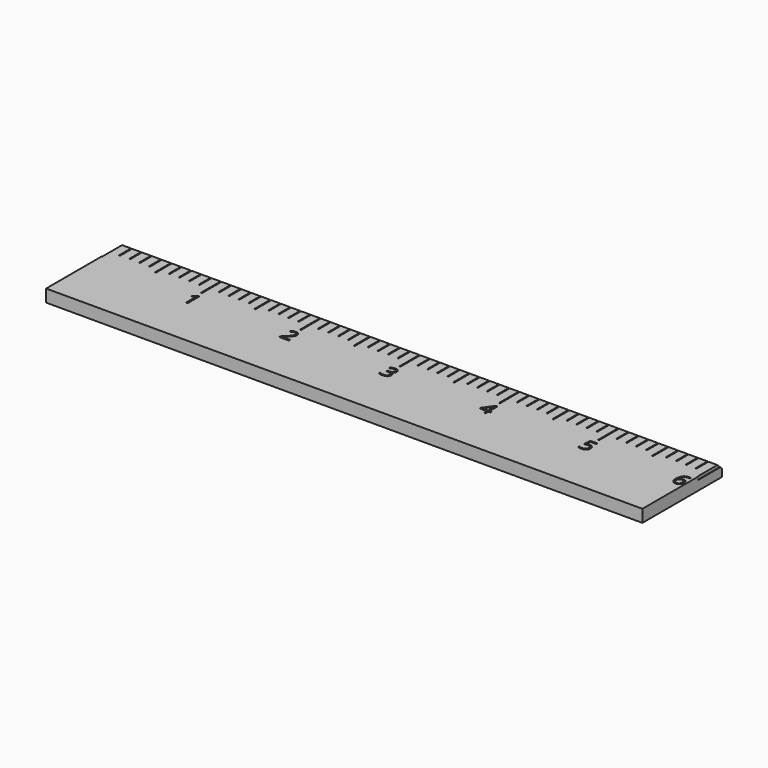
from build123d import *

# Parameters (mm, degrees)
F0_W          = 152.4
F0_H          = 25.4
F1_DEPTH      = 3.175
F2_W          = 0.254
F2_H          = 7.62
F2_H_2        = 5.08
F2_H_3        = 6.35
F3_TEXT_SIZE  = 5.2916666667
F4_DEPTH      = 0.762
F5_T3_DEPTH   = 8.8180747894
F5_T6_DEPTH   = 8.8180747894
F5_T9_DEPTH   = 8.8180747894
F5_T12_DEPTH  = 8.8180747894
F5_T15_DEPTH  = 8.8180747894
F5_T18_DEPTH  = 8.8180747894
F5_T21_DEPTH  = 8.8180747894
F5_T24_DEPTH  = 8.8180747894
F5_T27_DEPTH  = 8.8180747894
F5_T30_DEPTH  = 8.8180747894
F5_T33_DEPTH  = 8.8180747894
F5_T36_DEPTH  = 8.8180747894
F5_T39_DEPTH  = 8.8180747894
F5_T42_DEPTH  = 8.8180747894
F5_T45_DEPTH  = 8.8180747894
F5_T48_DEPTH  = 8.8180747894
F5_T51_DEPTH  = 8.8180747894
F5_T54_DEPTH  = 8.8180747894
F5_T57_DEPTH  = 8.8180747894
F5_T60_DEPTH  = 8.8180747894
F5_T63_DEPTH  = 8.8180747894
F5_T66_DEPTH  = 8.8180747894
F5_T69_DEPTH  = 8.8180747894
F5_T72_DEPTH  = 8.8180747894
F5_T75_DEPTH  = 8.8180747894
F5_T78_DEPTH  = 8.8180747894
F5_T81_DEPTH  = 8.8180747894
F5_T84_DEPTH  = 8.8180747894
F5_T87_DEPTH  = 8.8180747894
F5_T90_DEPTH  = 8.8180747894
F5_T93_DEPTH  = 8.8180747894
F5_T96_DEPTH  = 8.8180747894
F5_T99_DEPTH  = 8.8180747894
F5_T102_DEPTH = 8.8180747894
F5_T105_DEPTH = 8.8180747894
F5_T108_DEPTH = 8.8180747894
F5_T111_DEPTH = 8.8180747894
F5_T114_DEPTH = 8.8180747894
F5_T117_DEPTH = 8.8180747894
F5_T120_DEPTH = 8.8180747894
F5_T123_DEPTH = 8.8180747894
F5_T126_DEPTH = 8.8180747894
F5_T129_DEPTH = 8.8180747894
F5_T132_DEPTH = 8.8180747894
F5_T135_DEPTH = 8.8180747894
F5_T138_DEPTH = 8.8180747894
F5_T141_DEPTH = 8.8180747894
F5_T144_DEPTH = 8.8180747894
F5_T147_DEPTH = 8.8180747894
F5_T150_DEPTH = 8.8180747894
F5_T153_DEPTH = 8.8180747894
F5_T156_DEPTH = 8.8180747894
F5_T159_DEPTH = 8.8180747894
F5_T162_DEPTH = 8.8180747894
F5_T165_DEPTH = 8.8180747894
F5_T168_DEPTH = 8.8180747894
F5_T171_DEPTH = 8.8180747894
F5_T174_DEPTH = 8.8180747894
F5_T177_DEPTH = 8.8180747894
F5_T180_DEPTH = 8.8180747894


# Not quite as in the source:
# - a fillet or chamfer that OpenCascade refuses, or shapes differently, is made with other operations: its cross-section is extruded or revolved along the edge and cut away or added
# - Text() gives the source's letters only with a copy of the font that has no kerning and outlines rounded to 1/6400 em; it was checked with that copy


with BuildPart() as f1:
    # F0 (on Top) → F1 (new body)
    with BuildSketch(Plane.XY):
        Rectangle(F0_W, F0_H)
    extrude(amount=F1_DEPTH)

    # F2 (on face) + F3 (on face) → F4 (cut)
    with BuildSketch(Plane.XY.offset(3.175)):
        with Locations((-76.2, 8.89)):
            Rectangle(F2_W, F2_H)
        with Locations((-73.66, 10.16)):
            Rectangle(F2_W, F2_H_2)
        with Locations((-71.12, 10.16)):
            Rectangle(F2_W, F2_H_2)
        with Locations((-68.58, 10.16)):
            Rectangle(F2_W, F2_H_2)
        with Locations((-66.04, 10.16)):
            Rectangle(F2_W, F2_H_2)
        with Locations((-63.5, 9.525)):
            Rectangle(F2_W, F2_H_3)
        with Locations((-60.96, 10.16)):
            Rectangle(F2_W, F2_H_2)
        with Locations((-58.42, 10.16)):
            Rectangle(F2_W, F2_H_2)
        with Locations((-55.88, 10.16)):
            Rectangle(F2_W, F2_H_2)
        with Locations((-53.34, 10.16)):
            Rectangle(F2_W, F2_H_2)
        with Locations((-50.8, 8.89)):
            Rectangle(F2_W, F2_H)
        with Locations((-45.72, 10.16)):
            Rectangle(F2_W, F2_H_2)
        with Locations((-48.26, 10.16)):
            Rectangle(F2_W, F2_H_2)
        with Locations((-33.02, 10.16)):
            Rectangle(F2_W, F2_H_2)
        with Locations((-35.56, 10.16)):
            Rectangle(F2_W, F2_H_2)
        with Locations((-30.48, 10.16)):
            Rectangle(F2_W, F2_H_2)
        with Locations((-38.1, 9.525)):
            Rectangle(F2_W, F2_H_3)
        with Locations((-43.18, 10.16)):
            Rectangle(F2_W, F2_H_2)
        with Locations((-40.64, 10.16)):
            Rectangle(F2_W, F2_H_2)
        with Locations((-25.4, 8.89)):
            Rectangle(F2_W, F2_H)
        with Locations((-27.94, 10.16)):
            Rectangle(F2_W, F2_H_2)
        with Locations((-20.32, 10.16)):
            Rectangle(F2_W, F2_H_2)
        with Locations((-22.86, 10.16)):
            Rectangle(F2_W, F2_H_2)
        with Locations((-7.62, 10.16)):
            Rectangle(F2_W, F2_H_2)
        with Locations((-10.16, 10.16)):
            Rectangle(F2_W, F2_H_2)
        with Locations((-5.08, 10.16)):
            Rectangle(F2_W, F2_H_2)
        with Locations((-12.7, 9.525)):
            Rectangle(F2_W, F2_H_3)
        with Locations((-17.78, 10.16)):
            Rectangle(F2_W, F2_H_2)
        with Locations((-15.24, 10.16)):
            Rectangle(F2_W, F2_H_2)
        with Locations((0, 8.89)):
            Rectangle(F2_W, F2_H)
        with Locations((-2.54, 10.16)):
            Rectangle(F2_W, F2_H_2)
        with Locations((5.08, 10.16)):
            Rectangle(F2_W, F2_H_2)
        with Locations((2.54, 10.16)):
            Rectangle(F2_W, F2_H_2)
        with Locations((17.78, 10.16)):
            Rectangle(F2_W, F2_H_2)
        with Locations((15.24, 10.16)):
            Rectangle(F2_W, F2_H_2)
        with Locations((20.32, 10.16)):
            Rectangle(F2_W, F2_H_2)
        with Locations((12.7, 9.525)):
            Rectangle(F2_W, F2_H_3)
        with Locations((7.62, 10.16)):
            Rectangle(F2_W, F2_H_2)
        with Locations((10.16, 10.16)):
            Rectangle(F2_W, F2_H_2)
        with Locations((25.4, 8.89)):
            Rectangle(F2_W, F2_H)
        with Locations((22.86, 10.16)):
            Rectangle(F2_W, F2_H_2)
        with Locations((30.48, 10.16)):
            Rectangle(F2_W, F2_H_2)
        with Locations((27.94, 10.16)):
            Rectangle(F2_W, F2_H_2)
        with Locations((43.18, 10.16)):
            Rectangle(F2_W, F2_H_2)
        with Locations((40.64, 10.16)):
            Rectangle(F2_W, F2_H_2)
        with Locations((45.72, 10.16)):
            Rectangle(F2_W, F2_H_2)
        with Locations((38.1, 9.525)):
            Rectangle(F2_W, F2_H_3)
        with Locations((33.02, 10.16)):
            Rectangle(F2_W, F2_H_2)
        with Locations((35.56, 10.16)):
            Rectangle(F2_W, F2_H_2)
        with Locations((50.8, 8.89)):
            Rectangle(F2_W, F2_H)
        with Locations((48.26, 10.16)):
            Rectangle(F2_W, F2_H_2)
        with Locations((55.88, 10.16)):
            Rectangle(F2_W, F2_H_2)
        with Locations((53.34, 10.16)):
            Rectangle(F2_W, F2_H_2)
        with Locations((68.58, 10.16)):
            Rectangle(F2_W, F2_H_2)
        with Locations((66.04, 10.16)):
            Rectangle(F2_W, F2_H_2)
        with Locations((71.12, 10.16)):
            Rectangle(F2_W, F2_H_2)
        with Locations((63.5, 9.525)):
            Rectangle(F2_W, F2_H_3)
        with Locations((58.42, 10.16)):
            Rectangle(F2_W, F2_H_2)
        with Locations((60.96, 10.16)):
            Rectangle(F2_W, F2_H_2)
        with Locations((76.2, 8.89)):
            Rectangle(F2_W, F2_H)
        with Locations((73.66, 10.16)):
            Rectangle(F2_W, F2_H_2)
    with BuildSketch(Plane.XY.offset(3.175)):
        with Locations((-52.0221269531, 0)):
            Text('1', F3_TEXT_SIZE, font='Open Sans', text_align=(TextAlign.LEFT, TextAlign.BOTTOM))
        with Locations((-27.069438151, 0)):
            Text('2', F3_TEXT_SIZE, font='Open Sans', text_align=(TextAlign.LEFT, TextAlign.BOTTOM))
        with Locations((-1.6562089844, 0)):
            Text('3', F3_TEXT_SIZE, font='Open Sans', text_align=(TextAlign.LEFT, TextAlign.BOTTOM))
        with Locations((23.6416783854, 0)):
            Text('4', F3_TEXT_SIZE, font='Open Sans', text_align=(TextAlign.LEFT, TextAlign.BOTTOM))
        with Locations((49.1408971354, 0)):
            Text('5', F3_TEXT_SIZE, font='Open Sans', text_align=(TextAlign.LEFT, TextAlign.BOTTOM))
        with Locations((72.9624921875, 0)):
            Text('6', F3_TEXT_SIZE, font='Open Sans', text_align=(TextAlign.LEFT, TextAlign.BOTTOM))
    extrude(amount=-F4_DEPTH, mode=Mode.SUBTRACT)

    # F5: chamfer of 1.27 on 60 edges, made by hand


with BuildPart() as f5_tool1:
    # F5_s2 → F5_t3 (new body)
    with BuildSketch(Plane.YZ.offset(79.3390373947)):
        Polygon((11.43, 3.175), (12.7, 1.905), (12.7, 3.175), align=None)
    extrude(amount=-F5_T3_DEPTH)


with BuildPart() as f5_tool4:
    # F5_s5 → F5_t6 (new body)
    with BuildSketch(Plane.YZ.offset(-70.5209626053)):
        Polygon((11.43, 3.175), (12.7, 1.905), (12.7, 3.175), align=None)
    extrude(amount=-F5_T6_DEPTH)


with BuildPart() as f5_tool7:
    # F5_s8 → F5_t9 (new body)
    with BuildSketch(Plane.YZ.offset(-67.9809626053)):
        Polygon((11.43, 3.175), (12.7, 1.905), (12.7, 3.175), align=None)
    extrude(amount=-F5_T9_DEPTH)


with BuildPart() as f5_tool10:
    # F5_s11 → F5_t12 (new body)
    with BuildSketch(Plane.YZ.offset(-65.4409626053)):
        Polygon((11.43, 3.175), (12.7, 1.905), (12.7, 3.175), align=None)
    extrude(amount=-F5_T12_DEPTH)


with BuildPart() as f5_tool13:
    # F5_s14 → F5_t15 (new body)
    with BuildSketch(Plane.YZ.offset(-62.9009626053)):
        Polygon((11.43, 3.175), (12.7, 1.905), (12.7, 3.175), align=None)
    extrude(amount=-F5_T15_DEPTH)


with BuildPart() as f5_tool16:
    # F5_s17 → F5_t18 (new body)
    with BuildSketch(Plane.YZ.offset(-60.3609626053)):
        Polygon((11.43, 3.175), (12.7, 1.905), (12.7, 3.175), align=None)
    extrude(amount=-F5_T18_DEPTH)


with BuildPart() as f5_tool19:
    # F5_s20 → F5_t21 (new body)
    with BuildSketch(Plane.YZ.offset(-57.8209626053)):
        Polygon((11.43, 3.175), (12.7, 1.905), (12.7, 3.175), align=None)
    extrude(amount=-F5_T21_DEPTH)


with BuildPart() as f5_tool22:
    # F5_s23 → F5_t24 (new body)
    with BuildSketch(Plane.YZ.offset(-55.2809626053)):
        Polygon((11.43, 3.175), (12.7, 1.905), (12.7, 3.175), align=None)
    extrude(amount=-F5_T24_DEPTH)


with BuildPart() as f5_tool25:
    # F5_s26 → F5_t27 (new body)
    with BuildSketch(Plane.YZ.offset(-52.7409626053)):
        Polygon((11.43, 3.175), (12.7, 1.905), (12.7, 3.175), align=None)
    extrude(amount=-F5_T27_DEPTH)


with BuildPart() as f5_tool28:
    # F5_s29 → F5_t30 (new body)
    with BuildSketch(Plane.YZ.offset(-50.2009626053)):
        Polygon((11.43, 3.175), (12.7, 1.905), (12.7, 3.175), align=None)
    extrude(amount=-F5_T30_DEPTH)


with BuildPart() as f5_tool31:
    # F5_s32 → F5_t33 (new body)
    with BuildSketch(Plane.YZ.offset(-47.6609626053)):
        Polygon((11.43, 3.175), (12.7, 1.905), (12.7, 3.175), align=None)
    extrude(amount=-F5_T33_DEPTH)


with BuildPart() as f5_tool34:
    # F5_s35 → F5_t36 (new body)
    with BuildSketch(Plane.YZ.offset(-45.1209626053)):
        Polygon((11.43, 3.175), (12.7, 1.905), (12.7, 3.175), align=None)
    extrude(amount=-F5_T36_DEPTH)


with BuildPart() as f5_tool37:
    # F5_s38 → F5_t39 (new body)
    with BuildSketch(Plane.YZ.offset(-42.5809626053)):
        Polygon((11.43, 3.175), (12.7, 1.905), (12.7, 3.175), align=None)
    extrude(amount=-F5_T39_DEPTH)


with BuildPart() as f5_tool40:
    # F5_s41 → F5_t42 (new body)
    with BuildSketch(Plane.YZ.offset(-40.0409626053)):
        Polygon((11.43, 3.175), (12.7, 1.905), (12.7, 3.175), align=None)
    extrude(amount=-F5_T42_DEPTH)


with BuildPart() as f5_tool43:
    # F5_s44 → F5_t45 (new body)
    with BuildSketch(Plane.YZ.offset(-37.5009626053)):
        Polygon((11.43, 3.175), (12.7, 1.905), (12.7, 3.175), align=None)
    extrude(amount=-F5_T45_DEPTH)


with BuildPart() as f5_tool46:
    # F5_s47 → F5_t48 (new body)
    with BuildSketch(Plane.YZ.offset(-34.9609626053)):
        Polygon((11.43, 3.175), (12.7, 1.905), (12.7, 3.175), align=None)
    extrude(amount=-F5_T48_DEPTH)


with BuildPart() as f5_tool49:
    # F5_s50 → F5_t51 (new body)
    with BuildSketch(Plane.YZ.offset(-32.4209626053)):
        Polygon((11.43, 3.175), (12.7, 1.905), (12.7, 3.175), align=None)
    extrude(amount=-F5_T51_DEPTH)


with BuildPart() as f5_tool52:
    # F5_s53 → F5_t54 (new body)
    with BuildSketch(Plane.YZ.offset(-29.8809626053)):
        Polygon((11.43, 3.175), (12.7, 1.905), (12.7, 3.175), align=None)
    extrude(amount=-F5_T54_DEPTH)


with BuildPart() as f5_tool55:
    # F5_s56 → F5_t57 (new body)
    with BuildSketch(Plane.YZ.offset(-27.3409626053)):
        Polygon((11.43, 3.175), (12.7, 1.905), (12.7, 3.175), align=None)
    extrude(amount=-F5_T57_DEPTH)


with BuildPart() as f5_tool58:
    # F5_s59 → F5_t60 (new body)
    with BuildSketch(Plane.YZ.offset(-24.8009626053)):
        Polygon((11.43, 3.175), (12.7, 1.905), (12.7, 3.175), align=None)
    extrude(amount=-F5_T60_DEPTH)


with BuildPart() as f5_tool61:
    # F5_s62 → F5_t63 (new body)
    with BuildSketch(Plane.YZ.offset(-22.2609626053)):
        Polygon((11.43, 3.175), (12.7, 1.905), (12.7, 3.175), align=None)
    extrude(amount=-F5_T63_DEPTH)


with BuildPart() as f5_tool64:
    # F5_s65 → F5_t66 (new body)
    with BuildSketch(Plane.YZ.offset(-19.7209626053)):
        Polygon((11.43, 3.175), (12.7, 1.905), (12.7, 3.175), align=None)
    extrude(amount=-F5_T66_DEPTH)


with BuildPart() as f5_tool67:
    # F5_s68 → F5_t69 (new body)
    with BuildSketch(Plane.YZ.offset(-17.1809626053)):
        Polygon((11.43, 3.175), (12.7, 1.905), (12.7, 3.175), align=None)
    extrude(amount=-F5_T69_DEPTH)


with BuildPart() as f5_tool70:
    # F5_s71 → F5_t72 (new body)
    with BuildSketch(Plane.YZ.offset(-14.6409626053)):
        Polygon((11.43, 3.175), (12.7, 1.905), (12.7, 3.175), align=None)
    extrude(amount=-F5_T72_DEPTH)


with BuildPart() as f5_tool73:
    # F5_s74 → F5_t75 (new body)
    with BuildSketch(Plane.YZ.offset(-12.1009626053)):
        Polygon((11.43, 3.175), (12.7, 1.905), (12.7, 3.175), align=None)
    extrude(amount=-F5_T75_DEPTH)


with BuildPart() as f5_tool76:
    # F5_s77 → F5_t78 (new body)
    with BuildSketch(Plane.YZ.offset(-9.5609626053)):
        Polygon((11.43, 3.175), (12.7, 1.905), (12.7, 3.175), align=None)
    extrude(amount=-F5_T78_DEPTH)


with BuildPart() as f5_tool79:
    # F5_s80 → F5_t81 (new body)
    with BuildSketch(Plane.YZ.offset(-7.0209626053)):
        Polygon((11.43, 3.175), (12.7, 1.905), (12.7, 3.175), align=None)
    extrude(amount=-F5_T81_DEPTH)


with BuildPart() as f5_tool82:
    # F5_s83 → F5_t84 (new body)
    with BuildSketch(Plane.YZ.offset(-4.4809626053)):
        Polygon((11.43, 3.175), (12.7, 1.905), (12.7, 3.175), align=None)
    extrude(amount=-F5_T84_DEPTH)


with BuildPart() as f5_tool85:
    # F5_s86 → F5_t87 (new body)
    with BuildSketch(Plane.YZ.offset(-1.9409626053)):
        Polygon((11.43, 3.175), (12.7, 1.905), (12.7, 3.175), align=None)
    extrude(amount=-F5_T87_DEPTH)


with BuildPart() as f5_tool88:
    # F5_s89 → F5_t90 (new body)
    with BuildSketch(Plane.YZ.offset(0.5990373947)):
        Polygon((11.43, 3.175), (12.7, 1.905), (12.7, 3.175), align=None)
    extrude(amount=-F5_T90_DEPTH)


with BuildPart() as f5_tool91:
    # F5_s92 → F5_t93 (new body)
    with BuildSketch(Plane.YZ.offset(3.1390373947)):
        Polygon((11.43, 3.175), (12.7, 1.905), (12.7, 3.175), align=None)
    extrude(amount=-F5_T93_DEPTH)


with BuildPart() as f5_tool94:
    # F5_s95 → F5_t96 (new body)
    with BuildSketch(Plane.YZ.offset(5.6790373947)):
        Polygon((11.43, 3.175), (12.7, 1.905), (12.7, 3.175), align=None)
    extrude(amount=-F5_T96_DEPTH)


with BuildPart() as f5_tool97:
    # F5_s98 → F5_t99 (new body)
    with BuildSketch(Plane.YZ.offset(8.2190373947)):
        Polygon((11.43, 3.175), (12.7, 1.905), (12.7, 3.175), align=None)
    extrude(amount=-F5_T99_DEPTH)


with BuildPart() as f5_tool100:
    # F5_s101 → F5_t102 (new body)
    with BuildSketch(Plane.YZ.offset(10.7590373947)):
        Polygon((11.43, 3.175), (12.7, 1.905), (12.7, 3.175), align=None)
    extrude(amount=-F5_T102_DEPTH)


with BuildPart() as f5_tool103:
    # F5_s104 → F5_t105 (new body)
    with BuildSketch(Plane.YZ.offset(13.2990373947)):
        Polygon((11.43, 3.175), (12.7, 1.905), (12.7, 3.175), align=None)
    extrude(amount=-F5_T105_DEPTH)


with BuildPart() as f5_tool106:
    # F5_s107 → F5_t108 (new body)
    with BuildSketch(Plane.YZ.offset(15.8390373947)):
        Polygon((11.43, 3.175), (12.7, 1.905), (12.7, 3.175), align=None)
    extrude(amount=-F5_T108_DEPTH)


with BuildPart() as f5_tool109:
    # F5_s110 → F5_t111 (new body)
    with BuildSketch(Plane.YZ.offset(18.3790373947)):
        Polygon((11.43, 3.175), (12.7, 1.905), (12.7, 3.175), align=None)
    extrude(amount=-F5_T111_DEPTH)


with BuildPart() as f5_tool112:
    # F5_s113 → F5_t114 (new body)
    with BuildSketch(Plane.YZ.offset(20.9190373947)):
        Polygon((11.43, 3.175), (12.7, 1.905), (12.7, 3.175), align=None)
    extrude(amount=-F5_T114_DEPTH)


with BuildPart() as f5_tool115:
    # F5_s116 → F5_t117 (new body)
    with BuildSketch(Plane.YZ.offset(23.4590373947)):
        Polygon((11.43, 3.175), (12.7, 1.905), (12.7, 3.175), align=None)
    extrude(amount=-F5_T117_DEPTH)


with BuildPart() as f5_tool118:
    # F5_s119 → F5_t120 (new body)
    with BuildSketch(Plane.YZ.offset(25.9990373947)):
        Polygon((11.43, 3.175), (12.7, 1.905), (12.7, 3.175), align=None)
    extrude(amount=-F5_T120_DEPTH)


with BuildPart() as f5_tool121:
    # F5_s122 → F5_t123 (new body)
    with BuildSketch(Plane.YZ.offset(28.5390373947)):
        Polygon((11.43, 3.175), (12.7, 1.905), (12.7, 3.175), align=None)
    extrude(amount=-F5_T123_DEPTH)


with BuildPart() as f5_tool124:
    # F5_s125 → F5_t126 (new body)
    with BuildSketch(Plane.YZ.offset(31.0790373947)):
        Polygon((11.43, 3.175), (12.7, 1.905), (12.7, 3.175), align=None)
    extrude(amount=-F5_T126_DEPTH)


with BuildPart() as f5_tool127:
    # F5_s128 → F5_t129 (new body)
    with BuildSketch(Plane.YZ.offset(33.6190373947)):
        Polygon((11.43, 3.175), (12.7, 1.905), (12.7, 3.175), align=None)
    extrude(amount=-F5_T129_DEPTH)


with BuildPart() as f5_tool130:
    # F5_s131 → F5_t132 (new body)
    with BuildSketch(Plane.YZ.offset(36.1590373947)):
        Polygon((11.43, 3.175), (12.7, 1.905), (12.7, 3.175), align=None)
    extrude(amount=-F5_T132_DEPTH)


with BuildPart() as f5_tool133:
    # F5_s134 → F5_t135 (new body)
    with BuildSketch(Plane.YZ.offset(38.6990373947)):
        Polygon((11.43, 3.175), (12.7, 1.905), (12.7, 3.175), align=None)
    extrude(amount=-F5_T135_DEPTH)


with BuildPart() as f5_tool136:
    # F5_s137 → F5_t138 (new body)
    with BuildSketch(Plane.YZ.offset(41.2390373947)):
        Polygon((11.43, 3.175), (12.7, 1.905), (12.7, 3.175), align=None)
    extrude(amount=-F5_T138_DEPTH)


with BuildPart() as f5_tool139:
    # F5_s140 → F5_t141 (new body)
    with BuildSketch(Plane.YZ.offset(43.7790373947)):
        Polygon((11.43, 3.175), (12.7, 1.905), (12.7, 3.175), align=None)
    extrude(amount=-F5_T141_DEPTH)


with BuildPart() as f5_tool142:
    # F5_s143 → F5_t144 (new body)
    with BuildSketch(Plane.YZ.offset(46.3190373947)):
        Polygon((11.43, 3.175), (12.7, 1.905), (12.7, 3.175), align=None)
    extrude(amount=-F5_T144_DEPTH)


with BuildPart() as f5_tool145:
    # F5_s146 → F5_t147 (new body)
    with BuildSketch(Plane.YZ.offset(48.8590373947)):
        Polygon((11.43, 3.175), (12.7, 1.905), (12.7, 3.175), align=None)
    extrude(amount=-F5_T147_DEPTH)


with BuildPart() as f5_tool148:
    # F5_s149 → F5_t150 (new body)
    with BuildSketch(Plane.YZ.offset(51.3990373947)):
        Polygon((11.43, 3.175), (12.7, 1.905), (12.7, 3.175), align=None)
    extrude(amount=-F5_T150_DEPTH)


with BuildPart() as f5_tool151:
    # F5_s152 → F5_t153 (new body)
    with BuildSketch(Plane.YZ.offset(53.9390373947)):
        Polygon((11.43, 3.175), (12.7, 1.905), (12.7, 3.175), align=None)
    extrude(amount=-F5_T153_DEPTH)


with BuildPart() as f5_tool154:
    # F5_s155 → F5_t156 (new body)
    with BuildSketch(Plane.YZ.offset(56.4790373947)):
        Polygon((11.43, 3.175), (12.7, 1.905), (12.7, 3.175), align=None)
    extrude(amount=-F5_T156_DEPTH)


with BuildPart() as f5_tool157:
    # F5_s158 → F5_t159 (new body)
    with BuildSketch(Plane.YZ.offset(59.0190373947)):
        Polygon((11.43, 3.175), (12.7, 1.905), (12.7, 3.175), align=None)
    extrude(amount=-F5_T159_DEPTH)


with BuildPart() as f5_tool160:
    # F5_s161 → F5_t162 (new body)
    with BuildSketch(Plane.YZ.offset(61.5590373947)):
        Polygon((11.43, 3.175), (12.7, 1.905), (12.7, 3.175), align=None)
    extrude(amount=-F5_T162_DEPTH)


with BuildPart() as f5_tool163:
    # F5_s164 → F5_t165 (new body)
    with BuildSketch(Plane.YZ.offset(64.0990373947)):
        Polygon((11.43, 3.175), (12.7, 1.905), (12.7, 3.175), align=None)
    extrude(amount=-F5_T165_DEPTH)


with BuildPart() as f5_tool166:
    # F5_s167 → F5_t168 (new body)
    with BuildSketch(Plane.YZ.offset(66.6390373947)):
        Polygon((11.43, 3.175), (12.7, 1.905), (12.7, 3.175), align=None)
    extrude(amount=-F5_T168_DEPTH)


with BuildPart() as f5_tool169:
    # F5_s170 → F5_t171 (new body)
    with BuildSketch(Plane.YZ.offset(69.1790373947)):
        Polygon((11.43, 3.175), (12.7, 1.905), (12.7, 3.175), align=None)
    extrude(amount=-F5_T171_DEPTH)


with BuildPart() as f5_tool172:
    # F5_s173 → F5_t174 (new body)
    with BuildSketch(Plane.YZ.offset(71.7190373947)):
        Polygon((11.43, 3.175), (12.7, 1.905), (12.7, 3.175), align=None)
    extrude(amount=-F5_T174_DEPTH)


with BuildPart() as f5_tool175:
    # F5_s176 → F5_t177 (new body)
    with BuildSketch(Plane.YZ.offset(74.2590373947)):
        Polygon((11.43, 3.175), (12.7, 1.905), (12.7, 3.175), align=None)
    extrude(amount=-F5_T177_DEPTH)


with BuildPart() as f5_tool178:
    # F5_s179 → F5_t180 (new body)
    with BuildSketch(Plane.YZ.offset(76.7990373947)):
        Polygon((11.43, 3.175), (12.7, 1.905), (12.7, 3.175), align=None)
    extrude(amount=-F5_T180_DEPTH)


with BuildPart() as f1_1:
    add(f1.part)

    # F5_t181: cut F5_tool1, F5_tool4, F5_tool7, F5_tool10, F5_tool13, F5_tool16, F5_tool19, F5_tool22, F5_tool25, F5_tool28, F5_tool31, F5_tool34, F5_tool37, F5_tool40, F5_tool43, F5_tool46, F5_tool49, F5_tool52, F5_tool55, F5_tool58, F5_tool61, F5_tool64, F5_tool67, F5_tool70, F5_tool73, F5_tool76, F5_tool79, F5_tool82, F5_tool85, F5_tool88, F5_tool91, F5_tool94, F5_tool97, F5_tool100, F5_tool103, F5_tool106, F5_tool109, F5_tool112, F5_tool115, F5_tool118, F5_tool121, F5_tool124, F5_tool127, F5_tool130, F5_tool133, F5_tool136, F5_tool139, F5_tool142, F5_tool145, F5_tool148, F5_tool151, F5_tool154, F5_tool157, F5_tool160, F5_tool163, F5_tool166, F5_tool169, F5_tool172, F5_tool175, F5_tool178
    add([f5_tool1.part, f5_tool4.part, f5_tool7.part, f5_tool10.part, f5_tool13.part, f5_tool16.part, f5_tool19.part, f5_tool22.part, f5_tool25.part, f5_tool28.part, f5_tool31.part, f5_tool34.part, f5_tool37.part, f5_tool40.part, f5_tool43.part, f5_tool46.part, f5_tool49.part, f5_tool52.part, f5_tool55.part, f5_tool58.part, f5_tool61.part, f5_tool64.part, f5_tool67.part, f5_tool70.part, f5_tool73.part, f5_tool76.part, f5_tool79.part, f5_tool82.part, f5_tool85.part, f5_tool88.part, f5_tool91.part, f5_tool94.part, f5_tool97.part, f5_tool100.part, f5_tool103.part, f5_tool106.part, f5_tool109.part, f5_tool112.part, f5_tool115.part, f5_tool118.part, f5_tool121.part, f5_tool124.part, f5_tool127.part, f5_tool130.part, f5_tool133.part, f5_tool136.part, f5_tool139.part, f5_tool142.part, f5_tool145.part, f5_tool148.part, f5_tool151.part, f5_tool154.part, f5_tool157.part, f5_tool160.part, f5_tool163.part, f5_tool166.part, f5_tool169.part, f5_tool172.part, f5_tool175.part, f5_tool178.part], mode=Mode.SUBTRACT)


solid = f1_1.part
